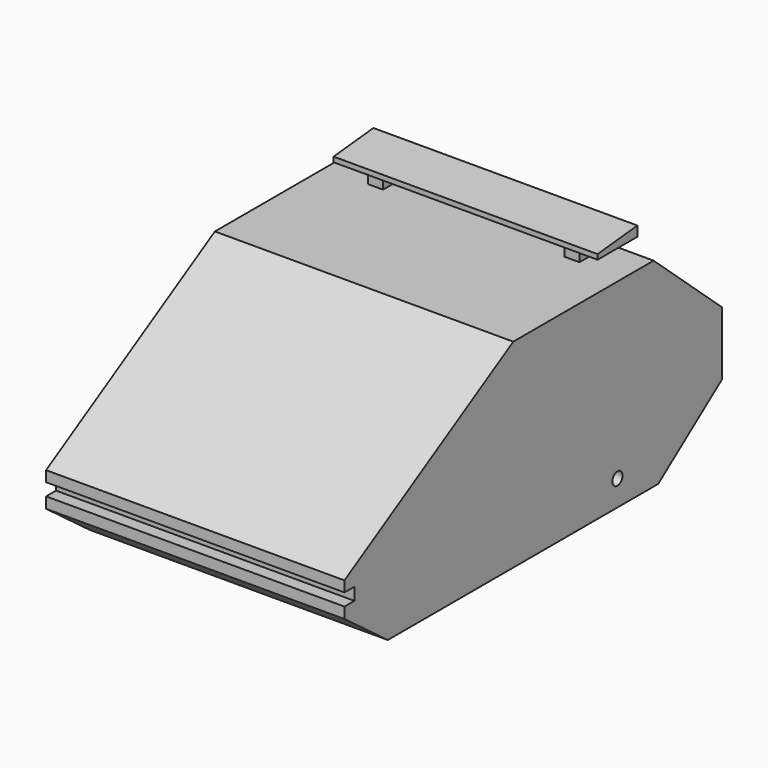
from build123d import *

# Parameters (mm, degrees)
F0_W      = 76.2
F0_H      = 127
F1_DEPTH  = 25.4
F2_W      = 76.2
F2_H      = 60.3884999398
F3_DEPTH  = 25.4
F5_DEPTH  = 25.4
F7_W      = 3.7973541766
F7_H      = 7.7133737504
F8_DEPTH  = 3.81
F9_W      = 67.4144178629
F9_H      = 12.7
F10_DEPTH = 2.54
F11_DEPTH = 25.4
F13_DEPTH = 119.38
F14_DEPTH = 157.988
F16_DEPTH = 160.7312
F18_DEPTH = 107.442
F19_DEPTH = 146.05
F22_DEPTH = 175.514
F23_R     = 1.6256
F24_DEPTH = 94.742
F25_W     = 85.8990699053
F25_H     = 3.175
F26_DEPTH = 3.175


with BuildPart() as f1:
    # F0 (on Top) → F1 (new body)
    with BuildSketch(Plane.XY):
        Rectangle(F0_W, F0_H)
    extrude(amount=F1_DEPTH)

    # F2 (on face) → F3 (join)
    with BuildSketch(Plane.XY.offset(25.4)):
        with Locations((0, -33.3057500301)):
            Rectangle(F2_W, F2_H)
    extrude(amount=F3_DEPTH)

    # F5 (add): a face of the model
    f5_faces = [f1.faces().sort_by_distance(p)[0] for p in [
        (0, 30.1942499699, 25.4),
    ]]
    extrude(f5_faces, amount=F5_DEPTH)

    # F7 (on face) → F8 (join)
    with BuildSketch(Plane.XY.offset(50.8)):
        with Locations((25.0877095386, 35.7790123671)):
            Rectangle(F7_W, F7_H)
        with Locations((-25.0877095386, 35.7790123671)):
            Rectangle(F7_W, F7_H)
    extrude(amount=F8_DEPTH)

    # F9 (on face) → F10 (join)
    with BuildSketch(Plane.XY.offset(54.61)):
        with Locations((0, 35.6483589858)):
            Rectangle(F9_W, F9_H)
    extrude(amount=F10_DEPTH)

    # F4 (on face) → F11 (join)
    with BuildSketch(Plane.YZ.offset(38.1)):
        Polygon((-63.5, 15.2083775029), (-3.1115000602, 50.8), (-63.5, 50.8), align=None)
    extrude(amount=F11_DEPTH)

    # F12 (on face) → F13 (cut)
    with BuildSketch(Plane.YZ.offset(63.5)):
        Polygon((-63.5, 50.8), (-63.5, 15.2083775029), (-3.1115000602, 50.8), align=None)
    extrude(amount=-F13_DEPTH, mode=Mode.SUBTRACT)

    # F6 (on face) → F14 (cut)
    with BuildSketch(Plane.YZ.offset(38.1)):
        Polygon((63.5, 50.8), (41.696511209, 50.8), (63.5, 31.4713791013), align=None)
    extrude(amount=-F14_DEPTH, mode=Mode.SUBTRACT)

    # F15 (on face) → F16 (cut)
    with BuildSketch(Plane.YZ.offset(33.7072089314)):
        Polygon((29.2983589858, 57.15), (29.2983589858, 55.88), (41.9983589858, 57.15), align=None)
    extrude(amount=-F16_DEPTH, mode=Mode.SUBTRACT)

    # F17 (on face) → F18 (cut)
    with BuildSketch(Plane.YZ.offset(38.1)):
        Polygon((-43.156321529, 0), (-63.5, 15.2083775029), (-63.5, 0), align=None)
    extrude(amount=-F18_DEPTH, mode=Mode.SUBTRACT)

    # F17 (on face) → F19 (cut)
    with BuildSketch(Plane.YZ.offset(38.1)):
        Polygon((63.5, 0), (63.5, 15.2083775029), (43.156321529, 0), align=None)
    extrude(amount=-F19_DEPTH, mode=Mode.SUBTRACT)

    # F21 (on face) → F22 (cut)
    with BuildSketch(Plane(origin=(-38.1, 0, 0), x_dir=(0, -1, 0), z_dir=(-1, 0, 0))):
        Polygon((67.4441531301, 13.2313063368), (56.999605149, 24.4063157588), (56.999605149, 6.1304802075), align=None)
    extrude(amount=-F22_DEPTH, mode=Mode.SUBTRACT)

    # F23 (on face) → F24 (cut)
    with BuildSketch(Plane.YZ.offset(38.1)):
        with Locations((30.1535148174, 6.5081091598)):
            Circle(F23_R)
    extrude(amount=-F24_DEPTH, mode=Mode.SUBTRACT)

    # F25 (on face) → F26 (cut)
    with BuildSketch(Plane.XZ.offset(56.999605149)):
        with Locations((0, 14.730398621)):
            Rectangle(F25_W, F25_H)
    extrude(amount=-F26_DEPTH, mode=Mode.SUBTRACT)


solid = f1.part
